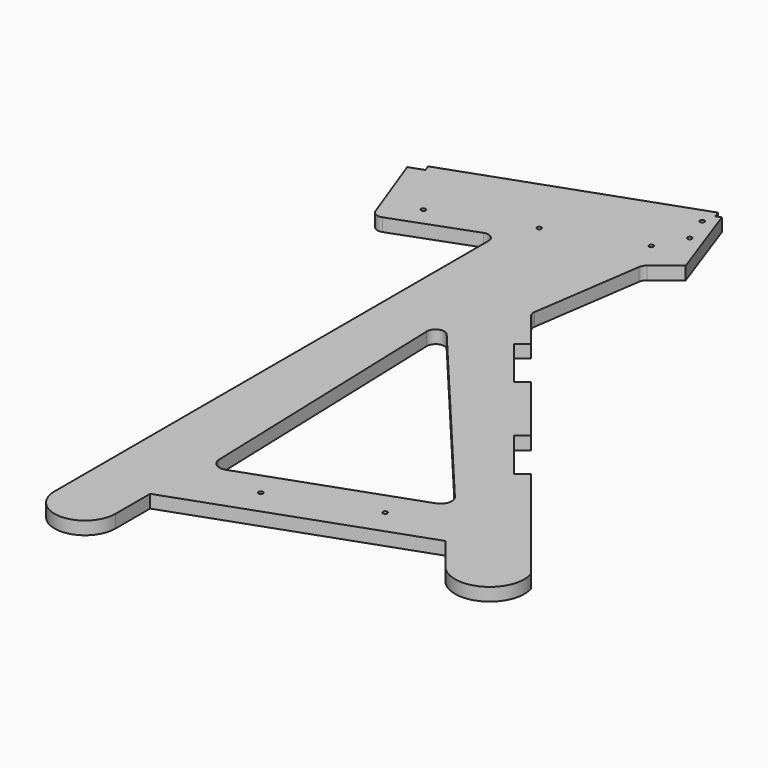
from build123d import *

# Parameters (mm, degrees)
F1_DEPTH = 19.05
F3_DEPTH = 9.525
F5_DEPTH = 9.525
F6_W     = 94.742
F6_H     = 19.05
F6_H_2   = 22.0252738774
F7_DEPTH = 19.558
F8_R     = 3.302
F9_DEPTH = 19.051


# Not quite as in the source:
# - a feature names something its author has since deleted; it is built from what else it names


with BuildPart() as f1:
    # F0 (on Top) → F1 (new body)
    with BuildSketch(Plane.XY):
        with BuildLine():
            Line((727.2677384075, 427.9083177516), (727.2677384075, -283.5772421425))
            ThreePointArc((727.2677384075, -283.5772421425), (771.8616098047, -328.1711135397), (816.4554812019, -283.5772421425))
            Line((816.4554812019, -283.5772421425), (816.4554812019, -220.0584400703))
            Line((816.4554812019, -220.0584400703), (1153.129473529, -100.186362138))
            Line((1153.129473529, -100.186362138), (1192.5444383312, -149.4502630935))
            ThreePointArc((1192.5444383312, -149.4502630935), (1256.128693756, -162.5951765711), (1280.8355912672, -102.5508970465))
            Line((1280.8355912672, -102.5508970465), (881.2480453078, 396.8848219998))
            ThreePointArc((881.2480453078, 396.8848219998), (878.9075846932, 401.4943033077), (878.5980767553, 406.6546597539))
            Line((878.5980767553, 406.6546597539), (902.2401524871, 568.497452094))
            ThreePointArc((902.2401524871, 568.497452094), (903.8120375637, 573.0182606597), (906.9455405898, 576.6362285378))
            Line((906.9455405898, 576.6362285378), (941.9003890149, 604.1852707886))
            Line((941.9003890149, 604.1852707886), (899.3018677789, 723.8279303566))
            Line((899.3018677789, 723.8279303566), (891.7270738587, 721.1309406639))
            Line((891.7270738587, 721.1309406639), (888.532184766, 730.1041401315))
            Line((888.532184766, 730.1041401315), (557.8398737201, 612.361827435))
            Line((557.8398737201, 612.361827435), (561.0347628128, 603.3886279674))
            Line((561.0347628128, 603.3886279674), (540.3738890749, 596.0323666485))
            Line((540.3738890749, 596.0323666485), (579.864860977, 488.7712220609))
            ThreePointArc((579.864860977, 488.7712220609), (586.4582383014, 481.6291726364), (596.1706516981, 481.2412028737))
            Line((596.1706516981, 481.2412028737), (710.1798391165, 523.2166417359))
            ThreePointArc((710.1798391165, 523.2166417359), (721.8328511307, 521.7154565085), (727.2677384075, 511.2987273493))
            Line((727.2677384075, 511.2987273493), (727.2677384075, 427.9083177516))
        make_face()
        with BuildLine():
            ThreePointArc((847.13107515, -119.4008734987), (832.2962861388, -117.4908698033), (825.0919590872, -104.3829809246))
            Line((825.0919590872, -104.3829809246), (812.2279623998, 291.9047427935))
            ThreePointArc((812.2279623998, 291.9047427935), (820.3847868922, 304.1789193457), (834.6503380579, 300.4798321914))
            Line((834.6503380579, 300.4798321914), (1093.5127410116, -8.0431735903))
            ThreePointArc((1093.5127410116, -8.0431735903), (1096.7972352344, -22.9844248457), (1086.4027687189, -34.2086823816))
            Line((1086.4027687189, -34.2086823816), (847.13107515, -119.4008734987))
        make_face(mode=Mode.SUBTRACT)
    extrude(amount=F1_DEPTH)

    # F2 (on face) → F3 (cut)
    with BuildSketch(Plane.XY):
        with BuildLine():
            ThreePointArc((844.1222933391, -166.9052020902), (847.3560158569, -170.6500208272), (852.2954479263, -170.9374917442))
            Line((852.2954479263, -170.9374917442), (1129.8610507564, -72.1108335167))
            ThreePointArc((1129.8610507564, -72.1108335167), (1133.425786756, -68.9382065458), (1133.77435322, -64.1788572139))
            Line((1133.77435322, -64.1788572139), (1131.667577719, -57.6492424267))
            ThreePointArc((1131.667577719, -57.6492424267), (1128.4338552012, -53.9044236898), (1123.4944231318, -53.6169527728))
            Line((1123.4944231318, -53.6169527728), (845.9288203018, -152.4436110002))
            ThreePointArc((845.9288203018, -152.4436110002), (842.3640843021, -155.6162379711), (842.0155178382, -160.3755873031))
            Line((842.0155178382, -160.3755873031), (844.1222933391, -166.9052020902))
        make_face()
    extrude(amount=F3_DEPTH, mode=Mode.SUBTRACT)

    # F4 (on face) → F5 (cut)
    with BuildSketch(Plane.XY):
        Polygon((579.9443241227, 521.366756094), (586.5044770697, 502.9417796404), (930.5357275267, 625.4329875525), (924.0377818739, 643.6832473584), (919.8348729601, 642.1868153078), (891.7270738587, 721.1309406639), (888.532184766, 730.1041401315), (870.0541627522, 723.6949228268), (901.3482962404, 635.8015951388), align=None)
    extrude(amount=F5_DEPTH, mode=Mode.SUBTRACT)

    # F6 (on face) → F7 (cut)
    with BuildSketch(Plane(origin=(730.9119602838, 584.7866009261, 0), x_dir=(-0.6247321984, 0.7808390873, 0), z_dir=(0.7808390873, 0.6247321984, 0))):
        with Locations((-357.8801403508, 9.525)):
            Rectangle(F6_W, F6_H)
        with Locations((-584.9891603508, 10.3152221296)):
            Rectangle(F6_W, F6_H_2)
    extrude(amount=-F7_DEPTH, mode=Mode.SUBTRACT)

    # F8 (on face) → F9 (cut, through all)
    with BuildSketch(Plane.XY):
        with Locations((902.6622274527, 660.6120369276)):
            Circle(F8_R)
        with Locations((887.9183335175, 702.107780571)):
            Circle(F8_R)
        with Locations((880.5389518172, 617.9122097817)):
            Circle(F8_R)
        with BuildLine():
            ThreePointArc((623.7483495144, 526.4827509324), (617.3838130375, 524.8132146381), (623.9396392041, 525.3751926427))
            ThreePointArc((623.9396392041, 525.3751926427), (623.8914653707, 525.9371706472), (623.7483495144, 526.4827509324))
        make_face()
        with BuildLine():
            ThreePointArc((756.0284718398, 572.4049919407), (752.1644938352, 575.6588181073), (749.6157615295, 571.2974336509))
            ThreePointArc((749.6157615295, 571.2974336509), (753.2884498444, 569.1511657741), (756.0284718398, 572.4049919407))
        make_face()
        with Locations((1055.4790926394, -88.2571151612)):
            Circle(F8_R)
        with Locations((913.5925848765, -138.7755124943)):
            Circle(F8_R)
    extrude(amount=F9_DEPTH, mode=Mode.SUBTRACT)


solid = f1.part
